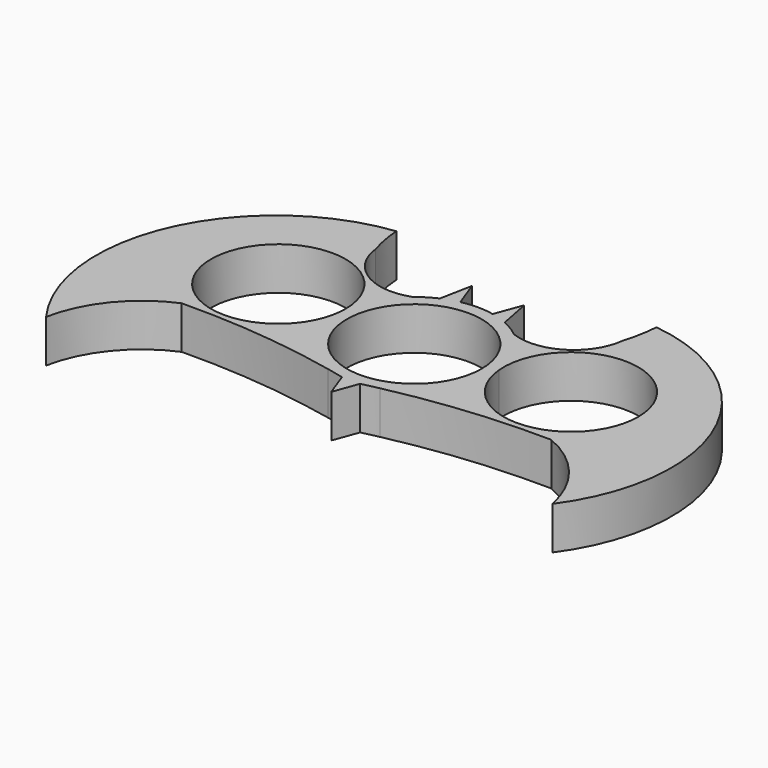
from build123d import *

# Parameters (mm, degrees)
F0_R     = 11
F1_DEPTH = 7


# Not quite as in the source:
# - a feature names something its author has since deleted; it is built from what else it names


with BuildPart() as f1:
    # F0 (on Top) → F1 (new body)
    with BuildSketch(Plane.XY):
        with BuildLine():
            ThreePointArc((8.2670150988, 10.0327693762), (6.6928166447, 10.8047053779), (5.3005300857, 11.87031511))
            ThreePointArc((5.3005300857, 11.87031511), (3.9954022113, 12.3708027698), (2.6440826014, 12.7282688217))
            ThreePointArc((2.6440826014, 12.7282688217), (0, 13), (-2.6440826014, 12.7282688217))
            ThreePointArc((-2.6440826014, 12.7282688217), (-3.9954022113, 12.3708027698), (-5.3005300857, 11.87031511))
            ThreePointArc((-5.3005300857, 11.87031511), (-6.6928166447, 10.8047053779), (-8.2670150988, 10.0327693762))
            ThreePointArc((-8.2670150988, 10.0327693762), (-11.5023304401, 6.0577549014), (-12.9498157312, 1.1411715589))
            ThreePointArc((-12.9498157312, 1.1411715589), (-10.91097159, -7.0675808423), (-4.2533323097, -12.2845091177))
            ThreePointArc((-4.2533323097, -12.2845091177), (-2.8648005364, -12.5913760507), (-1.4801854989, -12.9154578273))
            ThreePointArc((-1.4801854989, -12.9154578273), (0, -13), (1.4801854989, -12.9154578273))
            ThreePointArc((1.4801854989, -12.9154578273), (2.8648005364, -12.5913760507), (4.2533323097, -12.2845091177))
            ThreePointArc((4.2533323097, -12.2845091177), (10.5899320117, -7.5401153829), (13, 0))
            ThreePointArc((13, 0), (12.9870943447, 0.5791204378), (12.9484030029, 1.1570910404))
            ThreePointArc((12.9484030029, 1.1570910404), (11.4986046018, 6.0648241699), (8.2670150988, 10.0327693762))
        make_face()
        Circle(F0_R, mode=Mode.SUBTRACT)
        with BuildLine():
            ThreePointArc((2.6440826014, 12.7282688217), (3.9954022113, 12.3708027698), (5.3005300857, 11.87031511))
            Line((5.3005300857, 11.87031511), (4.2731994612, 17.1326149936))
            Line((4.2731994612, 17.1326149936), (2.6440826014, 12.7282688217))
        make_face()
        with BuildLine():
            ThreePointArc((8.2670150988, 10.0327693762), (6.8457077183, 11.0515286651), (5.3005300857, 11.87031511))
            ThreePointArc((5.3005300857, 11.87031511), (6.6928166447, 10.8047053779), (8.2670150988, 10.0327693762))
        make_face()
        with BuildLine():
            ThreePointArc((20.2180479346, 17.345385846), (16.0230615621, 10.7791515778), (8.2670150988, 10.0327693762))
            ThreePointArc((8.2670150988, 10.0327693762), (11.4986046018, 6.0648241699), (12.9484030029, 1.1570910404))
            ThreePointArc((12.9484030029, 1.1570910404), (12.9870943447, 0.5791204378), (13, 0))
            ThreePointArc((13, 0), (10.5899320117, -7.5401153829), (4.2533323097, -12.2845091177))
            ThreePointArc((4.2533323097, -12.2845091177), (17.1543822867, -10.2782846696), (30.1999320971, -9.7532540138))
            ThreePointArc((30.1999320971, -9.7532540138), (37.492259841, -15.2381838585), (41.3699261844, -23.4980992973))
            ThreePointArc((41.3699261844, -23.4980992973), (44.5988308489, 5.4669473875), (21.2553682043, 22.9163744996))
            ThreePointArc((21.2553682043, 22.9163744996), (20.8964882238, 20.1011290455), (20.2180479346, 17.345385846))
        make_face()
        with BuildLine():
            ThreePointArc((34.9047439829, 2.1361683247), (24.3947690942, -8.8529114999), (12.9484030029, 1.1570910404))
            ThreePointArc((12.9484030029, 1.1570910404), (23.4147188717, 13.1252481492), (34.9047439829, 2.1361683247))
        make_face(mode=Mode.SUBTRACT)
        with BuildLine():
            ThreePointArc((-5.3005300857, 11.87031511), (-3.9954022113, 12.3708027698), (-2.6440826014, 12.7282688217))
            Line((-2.6440826014, 12.7282688217), (-4.2731994612, 17.1326149936))
            Line((-4.2731994612, 17.1326149936), (-5.3005300857, 11.87031511))
        make_face()
        with BuildLine():
            ThreePointArc((-8.2670150988, 10.0327693762), (-6.6928166447, 10.8047053779), (-5.3005300857, 11.87031511))
            ThreePointArc((-5.3005300857, 11.87031511), (-6.8457077183, 11.0515286651), (-8.2670150988, 10.0327693762))
        make_face()
        with BuildLine():
            ThreePointArc((-12.9498157312, 1.1411715589), (-11.5023304401, 6.0577549014), (-8.2670150988, 10.0327693762))
            ThreePointArc((-8.2670150988, 10.0327693762), (-16.0230615621, 10.7791515778), (-20.2180479346, 17.345385846))
            ThreePointArc((-20.2180479346, 17.345385846), (-20.8964882238, 20.1011290455), (-21.2553682043, 22.9163744996))
            ThreePointArc((-21.2553682043, 22.9163744996), (-44.5988308489, 5.4669473875), (-41.3699261844, -23.4980992973))
            ThreePointArc((-41.3699261844, -23.4980992973), (-37.492259841, -15.2381838585), (-30.1999320971, -9.7532540138))
            ThreePointArc((-30.1999320971, -9.7532540138), (-17.1543822867, -10.2782846696), (-4.2533323097, -12.2845091177))
            ThreePointArc((-4.2533323097, -12.2845091177), (-10.91097159, -7.0675808423), (-12.9498157312, 1.1411715589))
        make_face()
        with BuildLine():
            ThreePointArc((-12.9073521155, 2.1067783052), (-12.917973147, 1.6235083115), (-12.9498157312, 1.1411715589))
            ThreePointArc((-12.9498157312, 1.1411715589), (-34.896731084, 2.5900482989), (-12.9073521155, 2.1067783052))
        make_face(mode=Mode.SUBTRACT)
        with BuildLine():
            Line((0, -16.953125596), (1.4801854989, -12.9154578273))
            ThreePointArc((1.4801854989, -12.9154578273), (0, -13), (-1.4801854989, -12.9154578273))
            Line((-1.4801854989, -12.9154578273), (0, -16.953125596))
        make_face()
    extrude(amount=F1_DEPTH)


solid = f1.part
